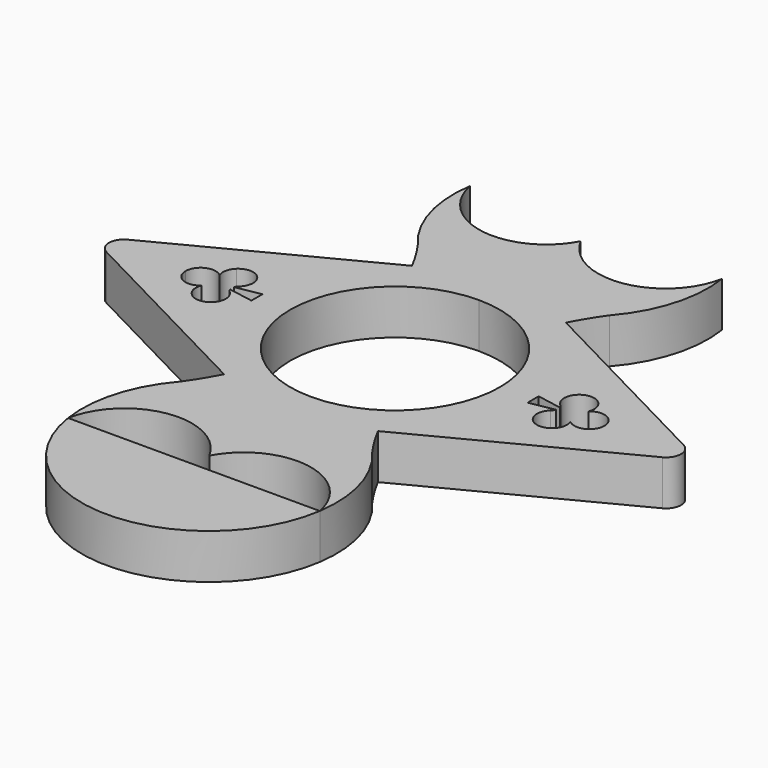
from build123d import *

# Parameters (mm, degrees)
F1_DEPTH    = 6
F2_T1_DEPTH = 25.2986514743
F4_DEPTH    = 6


# Not quite as in the source:
# - a fillet or chamfer that OpenCascade refuses, or shapes differently, is made with other operations: its cross-section is extruded or revolved along the edge and cut away or added


with BuildPart() as f1:
    # F0 (on Top) → F1 (new body)
    with BuildSketch(Plane.XY):
        with BuildLine():
            ThreePointArc((-5.8e-09, 14), (9.8994949346, 9.8994949386), (14, 0))
            ThreePointArc((14, 0), (9.8994949148, -9.8994949584), (-6.17e-08, -14))
            ThreePointArc((-6.17e-08, -14), (7.0324678211, -15.5227781451), (12.8050664705, -19.8183063588))
            ThreePointArc((12.8050664705, -19.8183063588), (11.4663069969, -17.796201056), (10.2746927153, -15.6840357719))
            Line((10.2746927153, -15.6840357719), (37.1157870048, -1.775761235))
            ThreePointArc((37.1157870048, -1.775761235), (38.195639171, 0), (37.1157870048, 1.775761235))
            Line((37.1157870048, 1.775761235), (10.2746927153, 15.6840357719))
            ThreePointArc((10.2746927153, 15.6840357719), (11.4663069969, 17.796201056), (12.8050664705, 19.8183063588))
            ThreePointArc((12.8050664705, 19.8183063588), (7.0324678466, 15.5227781567), (-5.8e-09, 14))
        make_face()
        with BuildLine():
            ThreePointArc((24.141058394, -3.738981755), (21.3116357879, -3.6427693993), (21.4131139219, -0.813530758))
            add(Edge.make_bspline(
                [(21.4131139219, -0.813530758), (21.5685270189, -0.6433130102), (21.7212531535, -0.4797257131), (21.771568805, -0.3264895931)],
                knots=[0, 0, 0, 0, 0.5764439926, 0.5764439926, 0.5764439926, 0.5764439926], degree=3))
            Line((21.771568805, -0.3264895931), (18.4447020292, -0.9186793468))
            Line((18.4447020292, -0.9186793468), (18.4447020292, 0.9186793468))
            Line((18.4447020292, 0.9186793468), (21.771568805, 0.3264895931))
            add(Edge.make_bspline(
                [(21.4131139219, 0.813530758), (21.5685270189, 0.6433130102), (21.7212531535, 0.4797257131), (21.771568805, 0.3264895931)],
                knots=[0, 0, 0, 0, 0.5764439926, 0.5764439926, 0.5764439926, 0.5764439926], degree=3))
            ThreePointArc((21.4131139219, 0.813530758), (21.3116357879, 3.6427693993), (24.141058394, 3.738981755))
            ThreePointArc((24.141058394, 3.738981755), (24.736062035, 2.6897370524), (24.6195059471, 1.4891711621))
            ThreePointArc((24.6195059471, 1.4891711621), (26.7807777011, 1.8396612496), (27.9680373117, 0))
            ThreePointArc((27.9680373117, 0), (26.7807777011, -1.8396612496), (24.6195059471, -1.4891711621))
            ThreePointArc((24.6195059471, -1.4891711621), (24.736062035, -2.6897370524), (24.141058394, -3.738981755))
        make_face(mode=Mode.SUBTRACT)
        with BuildLine():
            ThreePointArc((-6.17e-08, -14), (-14, 2.8e-08), (-5.8e-09, 14))
            ThreePointArc((-5.8e-09, 14), (-7.0324678518, 15.5227781591), (-12.8050664705, 19.8183063588))
            ThreePointArc((-12.8050664705, 19.8183063588), (-11.4663069969, 17.796201056), (-10.2746927153, 15.6840357719))
            Line((-10.2746927153, 15.6840357719), (-37.1157870048, 1.775761235))
            ThreePointArc((-37.1157870048, 1.775761235), (-38.195639171, 0), (-37.1157870048, -1.775761235))
            Line((-37.1157870048, -1.775761235), (-10.2746927153, -15.6840357719))
            ThreePointArc((-10.2746927153, -15.6840357719), (-11.4663069969, -17.796201056), (-12.8050664705, -19.8183063588))
            ThreePointArc((-12.8050664705, -19.8183063588), (-7.0324678773, -15.5227781707), (-6.17e-08, -14))
        make_face()
        with BuildLine():
            ThreePointArc((-24.6195059471, -1.4891711621), (-26.7807777011, -1.8396612496), (-27.9680373117, 0))
            ThreePointArc((-27.9680373117, 0), (-26.7807777011, 1.8396612496), (-24.6195059471, 1.4891711621))
            ThreePointArc((-24.6195059471, 1.4891711621), (-24.736062035, 2.6897370524), (-24.141058394, 3.738981755))
            ThreePointArc((-24.141058394, 3.738981755), (-21.3116357879, 3.6427693993), (-21.4131139219, 0.813530758))
            add(Edge.make_bspline(
                [(-21.4131139219, 0.813530758), (-21.5685270189, 0.6433130102), (-21.7212531535, 0.4797257131), (-21.771568805, 0.3264895931)],
                knots=[0, 0, 0, 0, 0.5764439926, 0.5764439926, 0.5764439926, 0.5764439926], degree=3))
            Line((-21.771568805, 0.3264895931), (-18.4447020292, 0.9186793468))
            Line((-18.4447020292, 0.9186793468), (-18.4447020292, -0.9186793468))
            Line((-18.4447020292, -0.9186793468), (-21.771568805, -0.3264895931))
            add(Edge.make_bspline(
                [(-21.4131139219, -0.813530758), (-21.5685270189, -0.6433130102), (-21.7212531535, -0.4797257131), (-21.771568805, -0.3264895931)],
                knots=[0, 0, 0, 0, 0.5764439926, 0.5764439926, 0.5764439926, 0.5764439926], degree=3))
            ThreePointArc((-21.4131139219, -0.813530758), (-21.3116357879, -3.6427693993), (-24.141058394, -3.738981755))
            ThreePointArc((-24.141058394, -3.738981755), (-24.736062035, -2.6897370524), (-24.6195059471, -1.4891711621))
        make_face(mode=Mode.SUBTRACT)
        with BuildLine():
            ThreePointArc((-12.8050664705, 19.8183063588), (-7.0324678518, 15.5227781591), (-5.8e-09, 14))
            ThreePointArc((-5.8e-09, 14), (7.0324678466, 15.5227781567), (12.8050664705, 19.8183063588))
            ThreePointArc((12.8050664705, 19.8183063588), (16.3226196216, 26.2489907715), (16.8056971277, 33.5629170979))
            ThreePointArc((16.8056971277, 33.5629170979), (9.3137334384, 26.3085555113), (0, 31))
            ThreePointArc((0, 31), (-9.3137334384, 26.3085555113), (-16.8056971277, 33.5629170979))
            ThreePointArc((-16.8056971277, 33.5629170979), (-16.3226196216, 26.2489907715), (-12.8050664705, 19.8183063588))
        make_face()
        with BuildLine():
            ThreePointArc((12.8050664705, -19.8183063588), (7.0324678211, -15.5227781451), (-6.17e-08, -14))
            ThreePointArc((-6.17e-08, -14), (-7.0324678773, -15.5227781707), (-12.8050664705, -19.8183063588))
            ThreePointArc((-12.8050664705, -19.8183063588), (-16.3226196216, -26.2489907715), (-16.8056971277, -33.5629170979))
            ThreePointArc((-16.8056971277, -33.5629170979), (-9.3137334384, -26.3085555113), (0, -31))
            ThreePointArc((0, -31), (9.3137334384, -26.3085555113), (16.8056971277, -33.5629170979))
            ThreePointArc((16.8056971277, -33.5629170979), (16.3226196216, -26.2489907715), (12.8050664705, -19.8183063588))
        make_face()
        with BuildLine():
            ThreePointArc((-37.1157870048, -1.775761235), (-38.195639171, 0), (-37.1157870048, 1.775761235))
            Line((-37.1157870048, 1.775761235), (-40.5427667225, 0))
            Line((-40.5427667225, 0), (-37.1157870048, -1.775761235))
        make_face()
        with BuildLine():
            Line((40.5427667225, 0), (37.1157870048, 1.775761235))
            ThreePointArc((37.1157870048, 1.775761235), (38.195639171, 0), (37.1157870048, -1.775761235))
            Line((37.1157870048, -1.775761235), (40.5427667225, 0))
        make_face()
    extrude(amount=F1_DEPTH)

    # F2: fillet of radius 2 on 2 edges, made by hand

    # F2_s2 → F2_t1 (cut)
    with BuildSketch(Plane.XY.offset(-9.6493257372)):
        with BuildLine():
            ThreePointArc((-37.1157870048, 1.775761235), (-38.195639171, 0), (-37.1157870048, -1.775761235))
            Line((-37.1157870048, -1.775761235), (-40.5427667225, 0))
            Line((-40.5427667225, 0), (-37.1157870048, 1.775761235))
        make_face()
        with BuildLine():
            ThreePointArc((37.1157870048, -1.775761235), (38.195639171, 0), (37.1157870048, 1.775761235))
            Line((37.1157870048, 1.775761235), (40.5427667225, 0))
            Line((40.5427667225, 0), (37.1157870048, -1.775761235))
        make_face()
    extrude(amount=F2_T1_DEPTH, mode=Mode.SUBTRACT)


with BuildPart() as f4:
    # F3 (on face) → F4 (new body)
    with BuildSketch(Plane(origin=(0, 0, 0), x_dir=(1, 0, 0), z_dir=(0, 0, -1))):
        with BuildLine():
            ThreePointArc((16.8056971277, 33.5629170979), (0, 48.046493252), (-16.8056971277, 33.5629170979))
            Line((-16.8056971277, 33.5629170979), (16.8056971277, 33.5629170979))
        make_face()
    extrude(amount=-F4_DEPTH)


solid = Compound([f1.part, f4.part])
